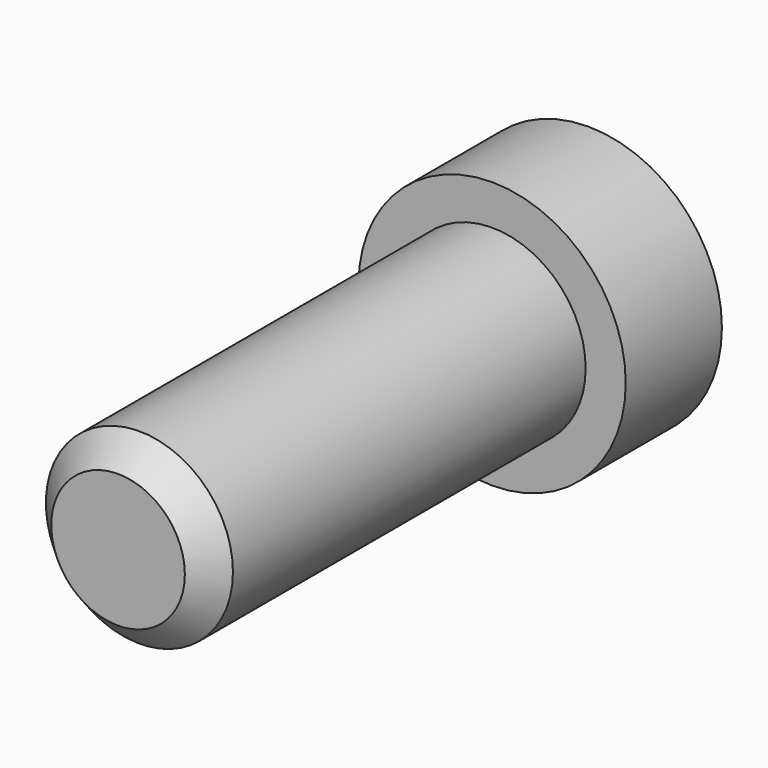
from build123d import *

# Parameters (mm, degrees)
F0_R     = 4.445
F1_DEPTH = 22.225
F2_R     = 6.35
F2_R_2   = 4.445
F3_DEPTH = 5.715
F4_SIZE  = 1.27


with BuildPart() as f1:
    # F0 (on Front) → F1 (new body)
    with BuildSketch(Plane.XZ):
        Circle(F0_R)
    extrude(amount=F1_DEPTH)

    # F2 (on face) → F3 (join)
    with BuildSketch(Plane(origin=(0, 0, 0), x_dir=(-1, 0, 0), z_dir=(0, 1, 0))):
        Circle(F2_R)
        Circle(F2_R_2, mode=Mode.SUBTRACT)
        Circle(F2_R_2)
    extrude(amount=F3_DEPTH)

    # F4
    f4_edges = [f1.edges().sort_by_distance(p)[0] for p in [
        (-4.445, -22.225, 0),
    ]]
    chamfer(f4_edges, length=F4_SIZE)


solid = f1.part
